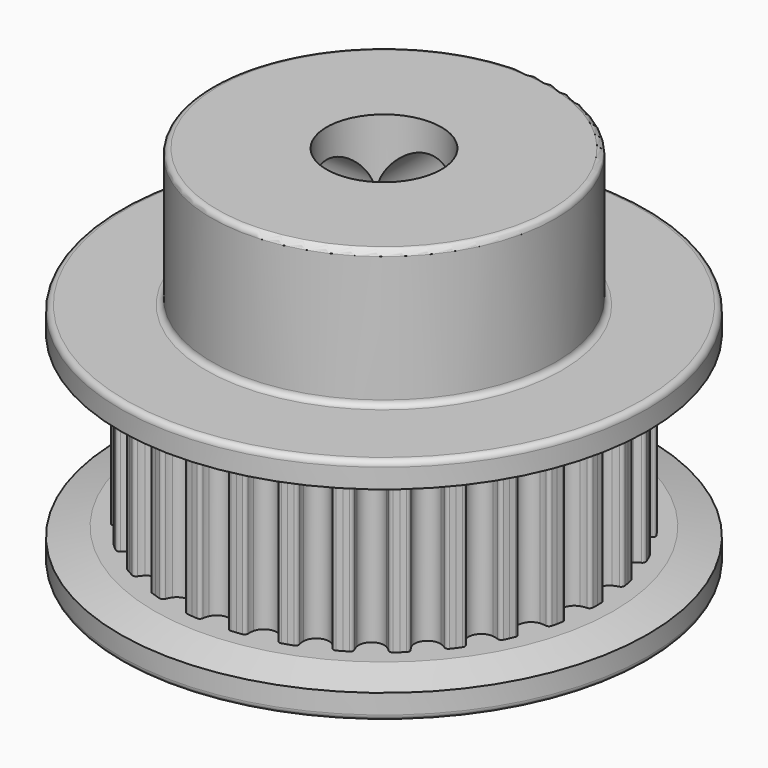
from build123d import *

# Parameters (mm, degrees)
F3_DEPTH    = 3.5
F4_COUNT    = 30
F5_R        = 11.5
F6_DEPTH    = 1.5
F7_R        = 11.5
F8_DEPTH    = 1.5
F9_R        = 7.5
F10_DEPTH   = 6
F11_R       = 2.5
F12_DEPTH   = 16.001
F13_R       = 1.75
F14_DEPTH   = 11.501
F15_R       = 1.75
F16_DEPTH   = 11.501
F17_SIZE2   = 0.4019237886
F17_SIZE    = 1.5
F17_2_SIZE2 = 0.4019237886
F17_2_SIZE  = 1.5
F18_R       = 0.25


# Not quite as in the source:
# - a feature names something its author has since deleted; it is built from what else it names


with BuildPart() as f3:
    # F2 (on Top) → F3 (new body, symmetric)
    with BuildSketch(Plane.XY):
        with BuildLine():
            ThreePointArc((0.5074445618, 8.8813827682), (0.3027155213, 8.640984901), (0, 8.5511604734))
            ThreePointArc((0, 8.5511604734), (-0.3027155213, 8.640984901), (-0.5074445618, 8.8813827682))
            ThreePointArc((-0.5074445618, 8.8813827682), (-0.5534043525, 9.0073298755), (-0.5821032352, 9.1382930394))
            ThreePointArc((-0.5821032352, 9.1382930394), (-0.6371721465, 9.2335496474), (-0.7424299509, 9.2655996234))
            ThreePointArc((-0.7424299509, 9.2655996234), (-0.8570922053, 9.255697249), (-0.9716230677, 9.2443759782))
            Line((-0.9716230677, 9.2443759782), (0, 0))
            Line((0, 0), (0.9716230677, 9.2443759782))
            ThreePointArc((0.9716230677, 9.2443759782), (0.8570922053, 9.255697249), (0.7424299509, 9.2655996234))
            ThreePointArc((0.7424299509, 9.2655996234), (0.6371721465, 9.2335496474), (0.5821032352, 9.1382930394))
            ThreePointArc((0.5821032352, 9.1382930394), (0.5534043525, 9.0073298755), (0.5074445618, 8.8813827682))
        make_face()
    extrude(amount=F3_DEPTH, both=True)

    # F4: F3 ×30 about axis
    f4_axis = Axis((0, 0, 0), (0, 0, -1))


with BuildPart() as f3_1:
    add(f3.part)
    for i in range(1, F4_COUNT):
        add(f3.part.rotate(f4_axis, i * 360 / F4_COUNT))

    # F5 (on face) → F6 (join)
    with BuildSketch(Plane(origin=(0, 0, -3.5), x_dir=(1, 0, 0), z_dir=(0, 0, -1))):
        Circle(F5_R)
    extrude(amount=F6_DEPTH)

    # F7 (on face) → F8 (join)
    with BuildSketch(Plane.XY.offset(3.5)):
        Circle(F7_R)
    extrude(amount=F8_DEPTH)

    # F9 (on face) → F10 (join)
    with BuildSketch(Plane.XY.offset(5)):
        Circle(F9_R)
    extrude(amount=F10_DEPTH)

    # F11 (on face) → F12 (cut, through all)
    with BuildSketch(Plane.XY.offset(11)):
        Circle(F11_R)
    extrude(amount=-F12_DEPTH, mode=Mode.SUBTRACT)

    # F13 (on Front) → F14 (cut, through all)
    with BuildSketch(Plane.XZ):
        with Locations((0, 8)):
            Circle(F13_R)
    extrude(amount=-F14_DEPTH, mode=Mode.SUBTRACT)

    # F15 (on Right) → F16 (cut, through all)
    with BuildSketch(Plane.YZ):
        with Locations((0, 8)):
            Circle(F15_R)
    extrude(amount=-F16_DEPTH, mode=Mode.SUBTRACT)

    # F17
    f17_edges = [f3_1.edges().sort_by_distance(p)[0] for p in [
        (-11.5, 0, -3.5),
    ]]
    f17_side = f3_1.faces().sort_by_distance((-11.174731, 0, -3.5))[0]
    chamfer(f17_edges, length=F17_SIZE, length2=F17_SIZE2, reference=f17_side)

    # F17#2
    f17_2_edges = [f3_1.edges().sort_by_distance(p)[0] for p in [
        (-11.5, 0, 3.5),
    ]]
    f17_2_side = f3_1.faces().sort_by_distance((-11.174731, 0, 3.5))[0]
    chamfer(f17_2_edges, length=F17_2_SIZE, length2=F17_2_SIZE2, reference=f17_2_side)

    # F18
    f18_edges = [f3_1.edges().sort_by_distance(p)[0] for p in [
        (-7.5, 0, 5),
        (-7.5, 0, 11),
        (-11.5, 0, 5),
        (-11.5, 0, -5),
    ]]
    fillet(f18_edges, radius=F18_R)


solid = f3_1.part
